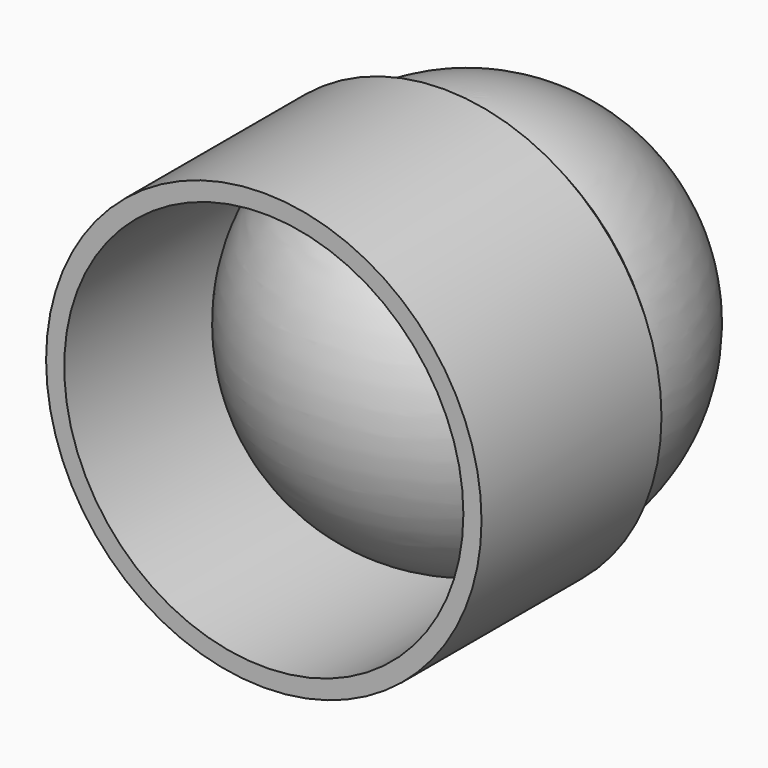
from build123d import *

# Parameters (mm, degrees)
F0_R     = 76.2
F0_R_2   = 69.85
F1_DEPTH = 88.9


# Not quite as in the source:
# - a fillet or chamfer that OpenCascade refuses, or shapes differently, is made with other operations: its cross-section is extruded or revolved along the edge and cut away or added


with BuildPart() as f1:
    # F0 (on Front) → F1 (new body)
    with BuildSketch(Plane.XZ):
        Circle(F0_R)
        Circle(F0_R_2, mode=Mode.SUBTRACT)
    extrude(amount=F1_DEPTH)

    # F4: chamfer of 10.16 on 1 edges, made by hand

    # F4_s1 → F4_t2 (revolve, cut)
    with BuildSketch(Plane.XY):
        Polygon((76.2, -10.16), (66.04, 0), (76.2, 0), align=None)
    revolve(axis=Axis((0, 0, 0), (0, -1, 0)), mode=Mode.SUBTRACT)


with BuildPart() as f3:
    # F2 (on Front) → F3 (revolve)
    with BuildSketch(Plane.XZ):
        with BuildLine():
            Line((0, -69.8497965932), (0, 69.8499903083))
            ThreePointArc((0, 69.8499903083), (-69.671833101, 9.68575e-05), (0, -69.8497965932))
        make_face()
    revolve(axis=Axis((0, 0, 9.68575e-05), (0, 0, -1)))


solid = Compound([f1.part, f3.part])
